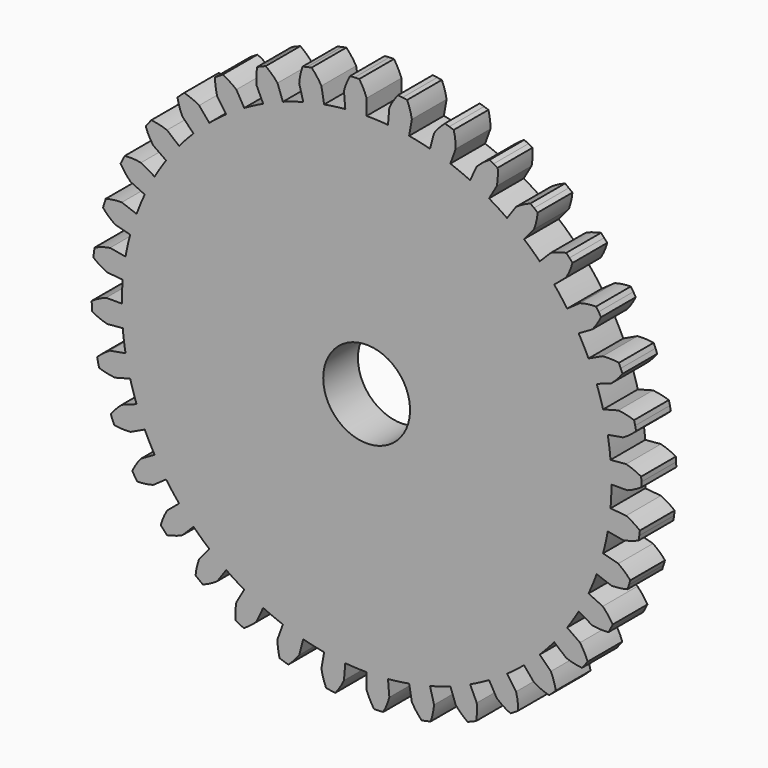
from build123d import *

# Parameters (mm, degrees)
F4_R     = 35.8022888519
F5_DEPTH = 6.35
F6_COUNT = 36
F9_D     = 12.7


with BuildPart() as f3:
    # F2 (on offset) → F3 section 0
    with BuildSketch(Plane.XZ.offset(6.35)):
        with BuildLine():
            ThreePointArc((-3.120375077, 35.6660503339), (-1.561673906, 35.7682130061), (0, 35.8022888519))
            Line((0, 35.8022888519), (0, 38.1))
            ThreePointArc((0, 38.1), (-0.4733366005, 39.1868313962), (-1.0780067417, 40.2064509535))
            Line((-1.0780067417, 40.2064509535), (-1.7546594511, 40.1883086861))
            Line((-1.7546594511, 40.1883086861), (-2.4303184955, 40.1474077472))
            ThreePointArc((-2.4303184955, 40.1474077472), (-2.9438219844, 39.0789676749), (-3.3206337987, 37.9550179973))
            Line((-3.3206337987, 37.9550179973), (-3.120375077, 35.6660503339))
        make_face()
    # F0 (on Front) → F3 section 1
    with BuildSketch(Plane.XZ):
        with BuildLine():
            ThreePointArc((-3.120375077, 35.6660503339), (-1.561673906, 35.7682130061), (0, 35.8022888519))
            Line((0, 35.8022888519), (0, 38.1))
            ThreePointArc((0, 38.1), (-0.4733366005, 39.1868313962), (-1.0780067417, 40.2064509535))
            Line((-1.0780067417, 40.2064509535), (-1.7546594511, 40.1883086861))
            Line((-1.7546594511, 40.1883086861), (-2.4303184955, 40.1474077472))
            ThreePointArc((-2.4303184955, 40.1474077472), (-2.9438219844, 39.0789676749), (-3.3206337987, 37.9550179973))
            Line((-3.3206337987, 37.9550179973), (-3.120375077, 35.6660503339))
        make_face()
    loft()

    # F4 (on offset) → F5 (join, through all)
    with BuildSketch(Plane.XZ.offset(6.35)):
        Circle(F4_R)
    extrude(amount=-F5_DEPTH)


with BuildPart() as f6_1:
    # F6: instance of F3
    add(f3.part.rotate(Axis((0, -6.35, 0), (0, -1, 0)), 1 * 360 / F6_COUNT))


with BuildPart() as f6_2:
    # F6: instance of F3
    add(f3.part.rotate(Axis((0, -6.35, 0), (0, -1, 0)), 2 * 360 / F6_COUNT))


with BuildPart() as f6_3:
    # F6: instance of F3
    add(f3.part.rotate(Axis((0, -6.35, 0), (0, -1, 0)), 3 * 360 / F6_COUNT))


with BuildPart() as f6_4:
    # F6: instance of F3
    add(f3.part.rotate(Axis((0, -6.35, 0), (0, -1, 0)), 4 * 360 / F6_COUNT))


with BuildPart() as f6_5:
    # F6: instance of F3
    add(f3.part.rotate(Axis((0, -6.35, 0), (0, -1, 0)), 5 * 360 / F6_COUNT))


with BuildPart() as f6_6:
    # F6: instance of F3
    add(f3.part.rotate(Axis((0, -6.35, 0), (0, -1, 0)), 6 * 360 / F6_COUNT))


with BuildPart() as f6_7:
    # F6: instance of F3
    add(f3.part.rotate(Axis((0, -6.35, 0), (0, -1, 0)), 7 * 360 / F6_COUNT))


with BuildPart() as f6_8:
    # F6: instance of F3
    add(f3.part.rotate(Axis((0, -6.35, 0), (0, -1, 0)), 8 * 360 / F6_COUNT))


with BuildPart() as f6_9:
    # F6: instance of F3
    add(f3.part.rotate(Axis((0, -6.35, 0), (0, -1, 0)), 9 * 360 / F6_COUNT))


with BuildPart() as f6_10:
    # F6: instance of F3
    add(f3.part.rotate(Axis((0, -6.35, 0), (0, -1, 0)), 10 * 360 / F6_COUNT))


with BuildPart() as f6_11:
    # F6: instance of F3
    add(f3.part.rotate(Axis((0, -6.35, 0), (0, -1, 0)), 11 * 360 / F6_COUNT))


with BuildPart() as f6_12:
    # F6: instance of F3
    add(f3.part.rotate(Axis((0, -6.35, 0), (0, -1, 0)), 12 * 360 / F6_COUNT))


with BuildPart() as f6_13:
    # F6: instance of F3
    add(f3.part.rotate(Axis((0, -6.35, 0), (0, -1, 0)), 13 * 360 / F6_COUNT))


with BuildPart() as f6_14:
    # F6: instance of F3
    add(f3.part.rotate(Axis((0, -6.35, 0), (0, -1, 0)), 14 * 360 / F6_COUNT))


with BuildPart() as f6_15:
    # F6: instance of F3
    add(f3.part.rotate(Axis((0, -6.35, 0), (0, -1, 0)), 15 * 360 / F6_COUNT))


with BuildPart() as f6_16:
    # F6: instance of F3
    add(f3.part.rotate(Axis((0, -6.35, 0), (0, -1, 0)), 16 * 360 / F6_COUNT))


with BuildPart() as f6_17:
    # F6: instance of F3
    add(f3.part.rotate(Axis((0, -6.35, 0), (0, -1, 0)), 17 * 360 / F6_COUNT))


with BuildPart() as f6_18:
    # F6: instance of F3
    add(f3.part.rotate(Axis((0, -6.35, 0), (0, -1, 0)), 18 * 360 / F6_COUNT))


with BuildPart() as f6_19:
    # F6: instance of F3
    add(f3.part.rotate(Axis((0, -6.35, 0), (0, -1, 0)), 19 * 360 / F6_COUNT))


with BuildPart() as f6_20:
    # F6: instance of F3
    add(f3.part.rotate(Axis((0, -6.35, 0), (0, -1, 0)), 20 * 360 / F6_COUNT))


with BuildPart() as f6_21:
    # F6: instance of F3
    add(f3.part.rotate(Axis((0, -6.35, 0), (0, -1, 0)), 21 * 360 / F6_COUNT))


with BuildPart() as f6_22:
    # F6: instance of F3
    add(f3.part.rotate(Axis((0, -6.35, 0), (0, -1, 0)), 22 * 360 / F6_COUNT))


with BuildPart() as f6_23:
    # F6: instance of F3
    add(f3.part.rotate(Axis((0, -6.35, 0), (0, -1, 0)), 23 * 360 / F6_COUNT))


with BuildPart() as f6_24:
    # F6: instance of F3
    add(f3.part.rotate(Axis((0, -6.35, 0), (0, -1, 0)), 24 * 360 / F6_COUNT))


with BuildPart() as f6_25:
    # F6: instance of F3
    add(f3.part.rotate(Axis((0, -6.35, 0), (0, -1, 0)), 25 * 360 / F6_COUNT))


with BuildPart() as f6_26:
    # F6: instance of F3
    add(f3.part.rotate(Axis((0, -6.35, 0), (0, -1, 0)), 26 * 360 / F6_COUNT))


with BuildPart() as f6_27:
    # F6: instance of F3
    add(f3.part.rotate(Axis((0, -6.35, 0), (0, -1, 0)), 27 * 360 / F6_COUNT))


with BuildPart() as f6_28:
    # F6: instance of F3
    add(f3.part.rotate(Axis((0, -6.35, 0), (0, -1, 0)), 28 * 360 / F6_COUNT))


with BuildPart() as f6_29:
    # F6: instance of F3
    add(f3.part.rotate(Axis((0, -6.35, 0), (0, -1, 0)), 29 * 360 / F6_COUNT))


with BuildPart() as f6_30:
    # F6: instance of F3
    add(f3.part.rotate(Axis((0, -6.35, 0), (0, -1, 0)), 30 * 360 / F6_COUNT))


with BuildPart() as f6_31:
    # F6: instance of F3
    add(f3.part.rotate(Axis((0, -6.35, 0), (0, -1, 0)), 31 * 360 / F6_COUNT))


with BuildPart() as f6_32:
    # F6: instance of F3
    add(f3.part.rotate(Axis((0, -6.35, 0), (0, -1, 0)), 32 * 360 / F6_COUNT))


with BuildPart() as f6_33:
    # F6: instance of F3
    add(f3.part.rotate(Axis((0, -6.35, 0), (0, -1, 0)), 33 * 360 / F6_COUNT))


with BuildPart() as f6_34:
    # F6: instance of F3
    add(f3.part.rotate(Axis((0, -6.35, 0), (0, -1, 0)), 34 * 360 / F6_COUNT))


with BuildPart() as f6_35:
    # F6: instance of F3
    add(f3.part.rotate(Axis((0, -6.35, 0), (0, -1, 0)), 35 * 360 / F6_COUNT))


with BuildPart() as f6_22_1:
    add(f6_22.part)

    # F7: union F3, F6_35, F6_34, F6_33, F6_32, F6_31, F6_30, F6_29, F6_28, F6_27, F6_1, F6_2, F6_3, F6_4, F6_5, F6_6, F6_7, F6_8, F6_9, F6_10, F6_26, F6_25, F6_24, F6_23, F6_21, F6_19, F6_18, F6_17, F6_16, F6_15, F6_14, F6_11, F6_12, F6_13, F6_20
    add(f3.part)
    add(f6_35.part)
    add(f6_34.part)
    add(f6_33.part)
    add(f6_32.part)
    add(f6_31.part)
    add(f6_30.part)
    add(f6_29.part)
    add(f6_28.part)
    add(f6_27.part)
    add(f6_1.part)
    add(f6_2.part)
    add(f6_3.part)
    add(f6_4.part)
    add(f6_5.part)
    add(f6_6.part)
    add(f6_7.part)
    add(f6_8.part)
    add(f6_9.part)
    add(f6_10.part)
    add(f6_26.part)
    add(f6_25.part)
    add(f6_24.part)
    add(f6_23.part)
    add(f6_21.part)
    add(f6_19.part)
    add(f6_18.part)
    add(f6_17.part)
    add(f6_16.part)
    add(f6_15.part)
    add(f6_14.part)
    add(f6_11.part)
    add(f6_12.part)
    add(f6_13.part)
    add(f6_20.part)

    # F9 (through all)
    with Locations(Plane.XZ.offset(6.35)):
        with Locations((0, 0)):
            Hole(F9_D / 2)


solid = f6_22_1.part
